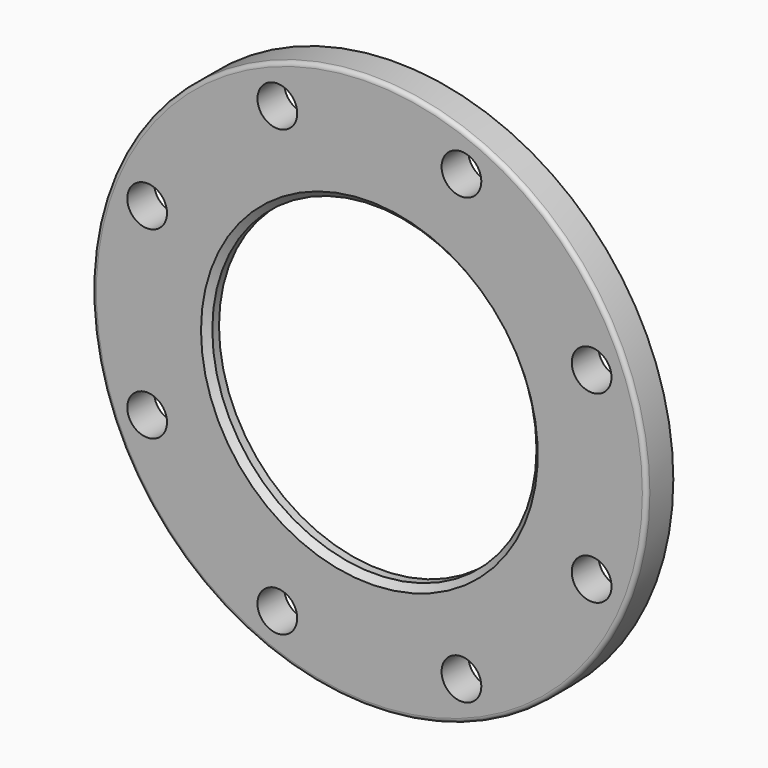
from build123d import *

# Parameters (mm, degrees)
F0_R     = 132.5
F0_R_2   = 9.5
F1_DEPTH = 18
F2_R     = 2
F3_R     = 132.5
F3_R_2   = 9.5
F3_R_3   = 103
F4_DEPTH = 2
F5_R     = 1.99999
F6_R     = 77.5
F7_DEPTH = 18.001
F6_R_2   = 92.6
F8_DEPTH = 11
F9_SIZE  = 3


# Not quite as in the source:
# - a fillet or chamfer is up to 0.001 mm smaller than in the source, because OpenCascade refuses the exact size


with BuildPart() as f1:
    # F0 (on Front) → F1 (new body)
    with BuildSketch(Plane.XZ):
        Circle(F0_R)
        with Locations((-44.008594722, -106.2461462388)):
            Circle(F0_R_2, mode=Mode.SUBTRACT)
        with Locations((-106.2461462388, -44.008594722)):
            Circle(F0_R_2, mode=Mode.SUBTRACT)
        with Locations((44.008594722, -106.2461462388)):
            Circle(F0_R_2, mode=Mode.SUBTRACT)
        with Locations((106.2461462388, -44.008594722)):
            Circle(F0_R_2, mode=Mode.SUBTRACT)
        with Locations((-106.2461462388, 44.008594722)):
            Circle(F0_R_2, mode=Mode.SUBTRACT)
        with Locations((-44.008594722, 106.2461462388)):
            Circle(F0_R_2, mode=Mode.SUBTRACT)
        with Locations((106.2461462388, 44.008594722)):
            Circle(F0_R_2, mode=Mode.SUBTRACT)
        with Locations((44.008594722, 106.2461462388)):
            Circle(F0_R_2, mode=Mode.SUBTRACT)
    extrude(amount=F1_DEPTH)

    # F2
    f2_edges = [f1.edges().sort_by_distance(p)[0] for p in [
        (-132.5, -18, 0),
    ]]
    fillet(f2_edges, radius=F2_R)

    # F3 (on face) → F4 (cut)
    with BuildSketch(Plane(origin=(0, 0, 0), x_dir=(-1, 0, 0), z_dir=(0, 1, 0))):
        Circle(F3_R)
        with Locations((-44.008594722, -106.2461462388)):
            Circle(F3_R_2, mode=Mode.SUBTRACT)
        with Locations((-106.2461462388, -44.008594722)):
            Circle(F3_R_2, mode=Mode.SUBTRACT)
        with Locations((44.008594722, -106.2461462388)):
            Circle(F3_R_2, mode=Mode.SUBTRACT)
        with Locations((106.2461462388, -44.008594722)):
            Circle(F3_R_2, mode=Mode.SUBTRACT)
        with Locations((-106.2461462388, 44.008594722)):
            Circle(F3_R_2, mode=Mode.SUBTRACT)
        with Locations((-44.008594722, 106.2461462388)):
            Circle(F3_R_2, mode=Mode.SUBTRACT)
        Circle(F3_R_3, mode=Mode.SUBTRACT)
        with Locations((106.2461462388, 44.008594722)):
            Circle(F3_R_2, mode=Mode.SUBTRACT)
        with Locations((44.008594722, 106.2461462388)):
            Circle(F3_R_2, mode=Mode.SUBTRACT)
    extrude(amount=-F4_DEPTH, mode=Mode.SUBTRACT)

    # F5 (radius 2 in the source; OpenCascade refuses exactly that, so slightly less here)
    f5_edges = [f1.edges().sort_by_distance(p)[0] for p in [
        (103, -2, 0),
    ]]
    fillet(f5_edges, radius=F5_R)

    # F6 (on face) → F7 (cut, through all)
    with BuildSketch(Plane(origin=(0, 0, 0), x_dir=(-1, 0, 0), z_dir=(0, 1, 0))):
        Circle(F6_R)
    extrude(amount=-F7_DEPTH, mode=Mode.SUBTRACT)

    # F6 (on face) → F8 (cut)
    with BuildSketch(Plane(origin=(0, 0, 0), x_dir=(-1, 0, 0), z_dir=(0, 1, 0))):
        Circle(F6_R_2)
        Circle(F6_R, mode=Mode.SUBTRACT)
    extrude(amount=-F8_DEPTH, mode=Mode.SUBTRACT)

    # F9
    f9_edges = [f1.edges().sort_by_distance(p)[0] for p in [
        (77.5, -18, 0),
    ]]
    chamfer(f9_edges, length=F9_SIZE)


solid = f1.part
